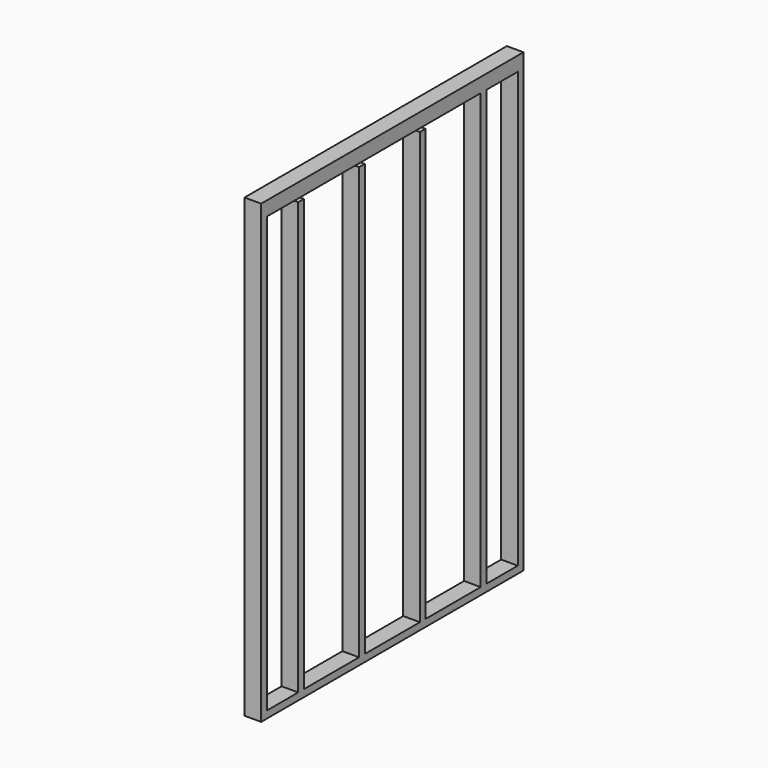
from build123d import *

# Parameters (mm, degrees)
F0_W     = 38.1
F0_H     = 2324.1
F0_W_2   = 1752.6
F0_H_2   = 38.1
F0_H_3   = 2306.102451545
F1_DEPTH = 88.9


with BuildPart() as f1:
    # F0 (on Right) → F1 (new body)
    with BuildSketch(Plane.YZ):
        Polygon((0, 38.1), (0, 0), (1752.6, 0), (1752.6, 38.1), (1714.5, 38.1), (1612.9, 38.1), (1504.95, 38.1), (1466.85, 38.1), (1098.55, 38.1), (1060.45, 38.1), (692.15, 38.1), (654.05, 38.1), (285.75, 38.1), (247.65, 38.1), (222.0338093996, 38.1), (215.9, 38.1), (177.8, 38.1), (38.1, 38.1), align=None)
        with Locations((19.05, 1200.15)):
            Rectangle(F0_W, F0_H)
        with Locations((1733.55, 1200.15)):
            Rectangle(F0_W, F0_H)
        Polygon((0, 2400.3), (0, 2362.2), (38.1, 2362.2), (177.8, 2362.2), (183.9338093996, 2362.2), (215.9, 2362.2), (1466.85, 2362.2), (1504.95, 2362.2), (1574.8, 2362.2), (1714.5, 2362.2), (1752.6, 2362.2), (1752.6, 2400.3), align=None)
        with Locations((876.3, 2419.35)):
            Rectangle(F0_W_2, F0_H_2)
        with Locations((1485.9, 1200.15)):
            Rectangle(F0_W, F0_H)
        with Locations((266.7, 1191.1512257725)):
            Rectangle(F0_W, F0_H_3)
        with Locations((1079.5, 1191.1512257725)):
            Rectangle(F0_W, F0_H_3)
        with Locations((673.1, 1191.1512257725)):
            Rectangle(F0_W, F0_H_3)
    extrude(amount=F1_DEPTH)


solid = f1.part
